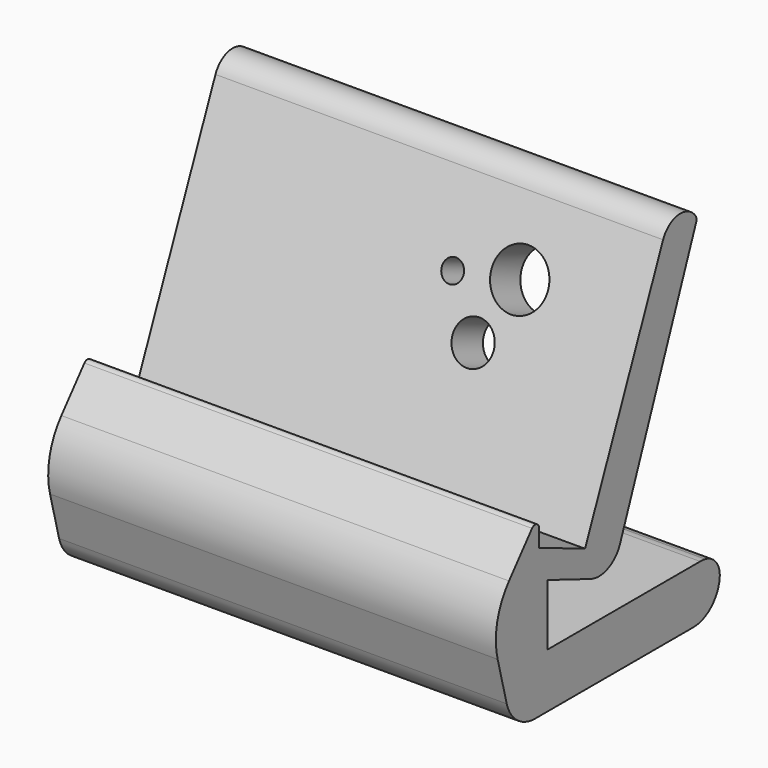
from build123d import *

# Parameters (mm, degrees)
F1_DEPTH     = 61
F2_R         = 9.670635699
F3_R         = 0.6712415125
F4_R         = 3.1919162273
F5_R         = 4.5432418233
F6_R         = 5
F7_R         = 3.8651714317
F7_R_2       = 1.4867583823
F7_R_3       = 2.8155117611
F8_DEPTH     = 25
F10_DEPTH    = 75.5
F11_R        = 3.8627416998
F12_T1_DEPTH = 73.5452662192
F13_R        = 3
F14_R        = 1


# Not quite as in the source:
# - a fillet or chamfer that OpenCascade refuses, or shapes differently, is made with other operations: its cross-section is extruded or revolved along the edge and cut away or added


with BuildPart() as f1:
    # F0 (on Right) → F1 (new body)
    with BuildSketch(Plane.YZ):
        with BuildLine():
            add(Edge.make_bspline(
                [(18.1424543803, -35.0754142348), (0, -24.5931053673), (21.0989990325, 0), (4.9723746061, 18.9487867674)],
                knots=[0, 0, 0, 0, 55.6063422209, 55.6063422209, 55.6063422209, 55.6063422209], degree=3))
            Line((4.9723746061, 18.9487867674), (-10.6166982745, -18.1424543803))
            Line((-10.6166982745, -18.1424543803), (-18.4527349874, -14.8490475373))
            Line((-18.4527349874, -14.8490475373), (-18.4527349874, -10.6166952334))
            Line((-18.4527349874, -10.6166952334), (-26.7433237145, -20.5614495141))
            Line((-26.7433237145, -20.5614495141), (-22.9804446479, -35.0754142348))
            Line((-22.9804446479, -35.0754142348), (18.1424543803, -35.0754142348))
        make_face()
    extrude(amount=F1_DEPTH)

    # F2
    f2_edges = [f1.edges().sort_by_distance(p)[0] for p in [
        (30.5, -26.743324, -20.56145),
    ]]
    fillet(f2_edges, radius=F2_R)

    # F3
    f3_edges = [f1.edges().sort_by_distance(p)[0] for p in [
        (30.5, -18.452735, -10.616695),
    ]]
    fillet(f3_edges, radius=F3_R)

    # F4
    f4_edges = [f1.edges().sort_by_distance(p)[0] for p in [
        (30.5, 4.972375, 18.948787),
    ]]
    fillet(f4_edges, radius=F4_R)

    # F5
    f5_edges = [f1.edges().sort_by_distance(p)[0] for p in [
        (30.5, 18.142454, -35.075414),
    ]]
    fillet(f5_edges, radius=F5_R)

    # F6
    f6_edges = [f1.edges().sort_by_distance(p)[0] for p in [
        (30.5, -22.980445, -35.075414),
    ]]
    fillet(f6_edges, radius=F6_R)

    # F7 (on face) → F8 (cut)
    with BuildSketch(Plane(origin=(0, -2.542493383, 1.0685842107), x_dir=(1, 0, 0), z_dir=(0, -0.9218866721, 0.3874596286))):
        with Locations((44.390194118, 4.044146277)):
            Circle(F7_R)
        with Locations((35.7474051416, 2.4390574545)):
            Circle(F7_R_2)
        with Locations((40.5626744032, -4.1047660634)):
            Circle(F7_R_3)
    extrude(amount=-F8_DEPTH, mode=Mode.SUBTRACT)

    # F9 (on face) → F10 (cut)
    with BuildSketch(Plane.YZ.offset(61)):
        Polygon((17.7633237159, 10.0974902644), (8.4745825412, 13.7160523356), (-6.0518267564, -23.5728081316), (-17.0180739519, -19.3007495805), (-17.0180739519, -27.6472643018), (21.4816201478, -27.6472643018), align=None)
    extrude(amount=-F10_DEPTH, mode=Mode.SUBTRACT)

    # F11
    f11_edges = [f1.edges().sort_by_distance(p)[0] for p in [
        (30.5, -6.051827, -23.572808),
    ]]
    fillet(f11_edges, radius=F11_R)

    # F12: fillet of radius 5 on 1 edges, made by hand

    # F12_s2 → F12_t1 (cut)
    with BuildSketch(Plane.YZ.offset(-6.2726331096)):
        with BuildLine():
            ThreePointArc((8.9937485165, -27.6472643018), (10.5238649897, -27.8871441795), (11.9071638019, -28.5837668704))
            Line((11.9071638019, -28.5837668704), (11.9654321077, -28.5024969218))
            ThreePointArc((11.9654321077, -28.5024969218), (11.7885278554, -28.0794589932), (11.5959390896, -27.6108577379))
            Line((11.5959390896, -27.6108577379), (11.5028017603, -27.5472643018))
            Line((11.5028017603, -27.5472643018), (8.9937485165, -27.5472643018))
            Line((8.9937485165, -27.5472643018), (8.9937485165, -27.6472643018))
        make_face()
    extrude(amount=F12_T1_DEPTH, mode=Mode.SUBTRACT)

    # F13
    f13_edges = [f1.edges().sort_by_distance(p)[0] for p in [
        (30.5, 11.907164, -28.583767),
    ]]
    fillet(f13_edges, radius=F13_R)

    # F14
    f14_edges = [f1.edges().sort_by_distance(p)[0] for p in [
        (30.5, 8.474583, 13.716052),
    ]]
    fillet(f14_edges, radius=F14_R)


solid = f1.part
